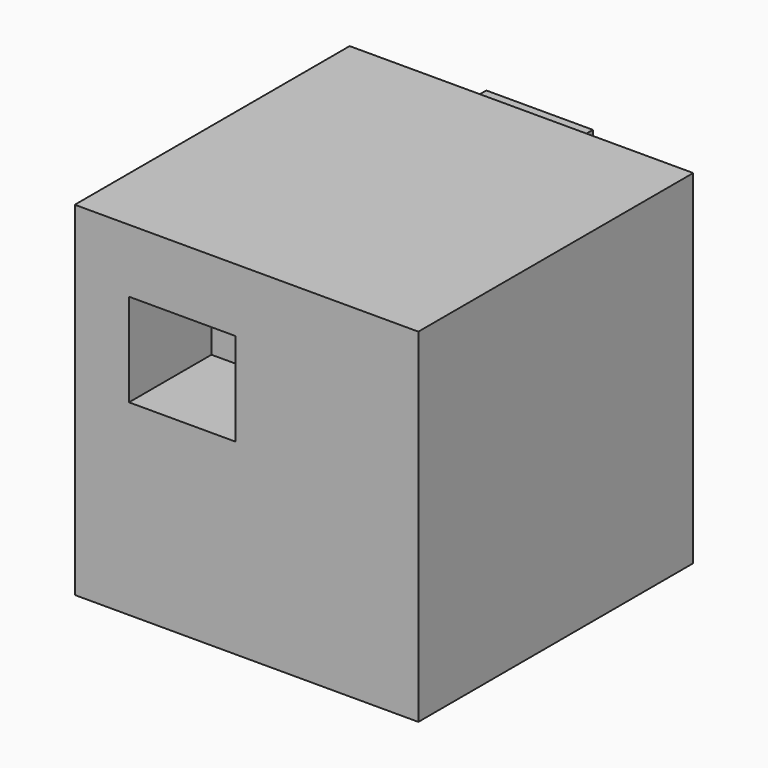
from build123d import *

# Parameters (mm, degrees)
F1_W     = 254
F1_H     = 254
F2_DEPTH = 127
F3_W     = 78.8055062294
F3_H     = 68.7452331185
F4_DEPTH = 76.2
F5_W     = 78.8055062294
F5_H     = 68.7452331185
F6_DEPTH = 76.2


# Not quite as in the source:
# - a variable given as a bare number and used for a length is read in inches; the dataset says mm whatever the document's units were


with BuildPart() as f2:
    # F1 (on Front) → F2 (new body, symmetric)
    with BuildSketch(Plane.XZ):
        with Locations((103.069830358, 103.7981395125)):
            Rectangle(F1_W, F1_H)
    extrude(amount=F2_DEPTH, both=True)

    # F3 (on face) → F4 (cut)
    with BuildSketch(Plane.XZ.offset(127)):
        with Locations((55.5568262935, 149.6073119342)):
            Rectangle(F3_W, F3_H)
    extrude(amount=-F4_DEPTH, mode=Mode.SUBTRACT)


with BuildPart() as f6:
    # F5 (on face) → F6 (new body)
    with BuildSketch(Plane(origin=(0, 127, 0), x_dir=(-1, 0, 0), z_dir=(0, 1, 0))):
        with Locations((-55.5568262935, 149.6073119342)):
            Rectangle(F5_W, F5_H)
    extrude(amount=F6_DEPTH)


solid = Compound([f2.part, f6.part])
